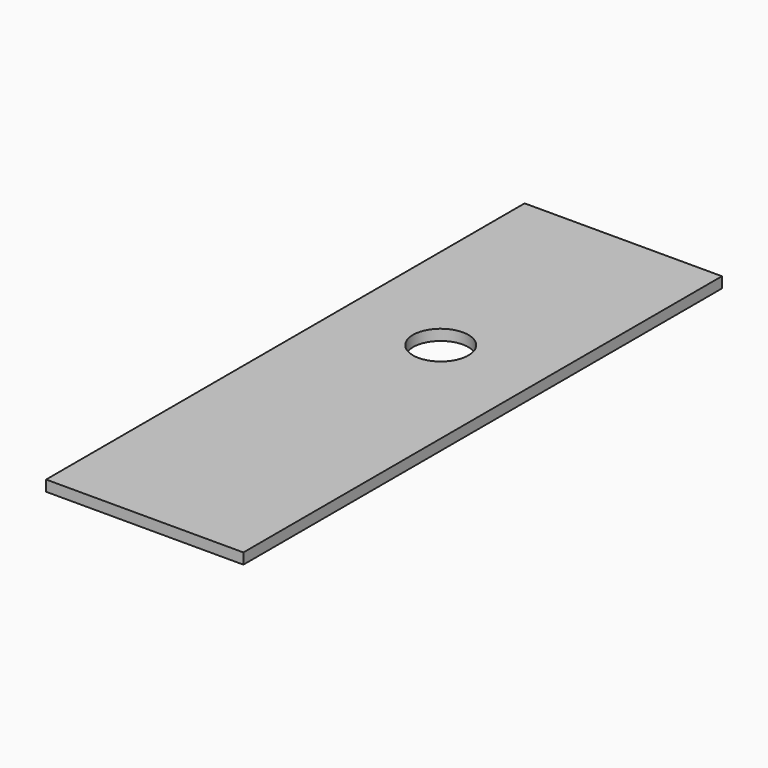
from build123d import *

# Parameters (mm, degrees)
F0_W     = 812.8
F0_H     = 2463.8
F1_DEPTH = 44.45
F3_D     = 228.6
F4_W     = 812.8
F4_H     = 50.8
F5_DEPTH = 3.429


# Not quite as in the source:
# - a feature names something its author has since deleted; it is built from what else it names


with BuildPart() as f1:
    # F0 (on Top) → F1 (new body)
    with BuildSketch(Plane.XY):
        with Locations((406.4, 1231.9)):
            Rectangle(F0_W, F0_H)
    extrude(amount=F1_DEPTH)

    # F3 (through all)
    with Locations(Plane.XY.offset(44.45)):
        with Locations((406.4, 1524)):
            Hole(F3_D / 2)

    # F4 (on face) → F5 (join)
    with BuildSketch(Plane.XY.offset(44.45)):
        with Locations((406.4, 2133.6)):
            Rectangle(F4_W, F4_H)
        with Locations((406.4, 2032)):
            Rectangle(F4_W, F4_H)
        with Locations((406.4, 1930.4)):
            Rectangle(F4_W, F4_H)
        with Locations((406.4, 1828.8)):
            Rectangle(F4_W, F4_H)
        with Locations((406.4, 1727.2)):
            Rectangle(F4_W, F4_H)
        with BuildLine():
            Line((0, 1549.4), (0, 1498.6))
            Line((0, 1498.6), (256.1315735093, 1498.6))
            ThreePointArc((256.1315735093, 1498.6), (254, 1524), (256.1315735093, 1549.4))
            Line((256.1315735093, 1549.4), (0, 1549.4))
        make_face()
        with BuildLine():
            Line((556.6684264907, 1498.6), (812.8, 1498.6))
            Line((812.8, 1498.6), (812.8, 1549.4))
            Line((812.8, 1549.4), (556.6684264907, 1549.4))
            ThreePointArc((556.6684264907, 1549.4), (558.2661716729, 1536.7446420666), (558.8, 1524))
            ThreePointArc((558.8, 1524), (558.2661716729, 1511.2553579334), (556.6684264907, 1498.6))
        make_face()
        with BuildLine():
            Line((490.642269675, 1397), (812.8, 1397))
            Line((812.8, 1397), (812.8, 1447.8))
            Line((812.8, 1447.8), (538.3822715367, 1447.8))
            ThreePointArc((538.3822715367, 1447.8), (517.455945611, 1419.6336407436), (490.642269675, 1397))
        make_face()
        with Locations((406.4, 1320.8)):
            Rectangle(F4_W, F4_H)
        Polygon((0, 1231.9), (0, 1193.8), (812.8, 1193.8), (812.8, 1231.9), (812.8, 1244.6), (0, 1244.6), align=None)
        with Locations((406.4, 1117.6)):
            Rectangle(F4_W, F4_H)
        with Locations((406.4, 1016)):
            Rectangle(F4_W, F4_H)
        with Locations((406.4, 914.4)):
            Rectangle(F4_W, F4_H)
        with Locations((406.4, 812.8)):
            Rectangle(F4_W, F4_H)
        with Locations((406.4, 711.2)):
            Rectangle(F4_W, F4_H)
        with Locations((406.4, 609.6)):
            Rectangle(F4_W, F4_H)
        with Locations((406.4, 508)):
            Rectangle(F4_W, F4_H)
        with Locations((406.4, 406.4)):
            Rectangle(F4_W, F4_H)
        with Locations((406.4, 304.8)):
            Rectangle(F4_W, F4_H)
        with Locations((406.4, 203.2)):
            Rectangle(F4_W, F4_H)
        with BuildLine():
            Line((538.3822715367, 1600.2), (812.8, 1600.2))
            Line((812.8, 1600.2), (812.8, 1651))
            Line((812.8, 1651), (490.642269675, 1651))
            ThreePointArc((490.642269675, 1651), (517.455945611, 1628.3663592564), (538.3822715367, 1600.2))
        make_face()
        with BuildLine():
            Line((0, 1447.8), (0, 1397))
            Line((0, 1397), (322.157730325, 1397))
            ThreePointArc((322.157730325, 1397), (295.344054389, 1419.6336407436), (274.4177284633, 1447.8))
            Line((274.4177284633, 1447.8), (0, 1447.8))
        make_face()
        with BuildLine():
            Line((0, 1651), (0, 1600.2))
            Line((0, 1600.2), (274.4177284633, 1600.2))
            ThreePointArc((274.4177284633, 1600.2), (295.344054389, 1628.3663592564), (322.157730325, 1651))
            Line((322.157730325, 1651), (0, 1651))
        make_face()
    extrude(amount=-F5_DEPTH)


solid = f1.part
